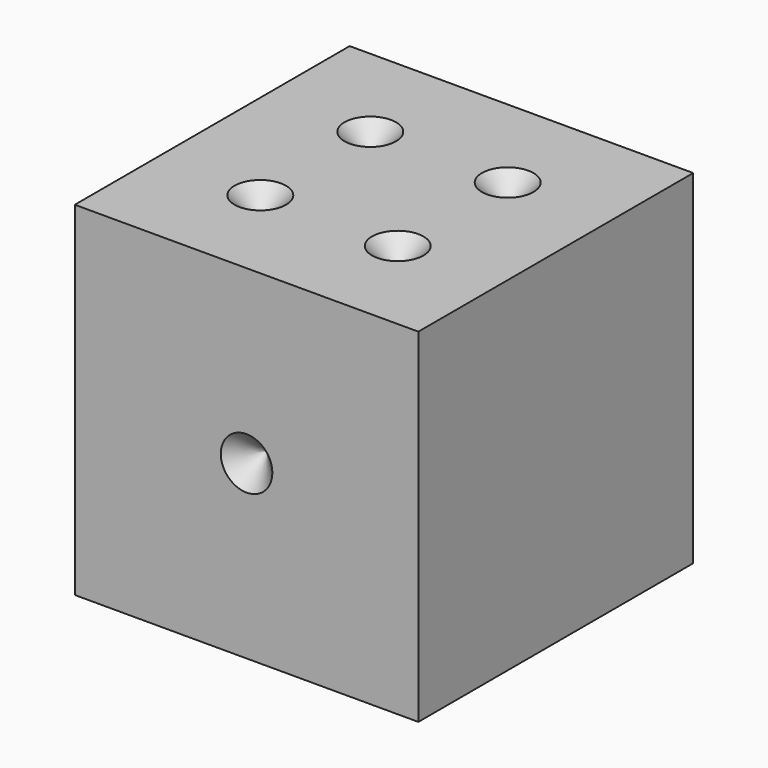
from build123d import *

# Parameters (mm, degrees)
F0_W     = 20
F0_H     = 20
F1_DEPTH = 20
F2_R     = 1.5
F3_DEPTH = 1.5
F4_R     = 1.5
F5_DEPTH = 1.5
F6_SIZE  = 1.49999


# Not quite as in the source:
# - a fillet or chamfer is up to 0.001 mm smaller than in the source, because OpenCascade refuses the exact size


with BuildPart() as f1:
    # F0 (on Top) → F1 (new body)
    with BuildSketch(Plane.XY):
        with Locations((10, 10)):
            Rectangle(F0_W, F0_H)
    extrude(amount=F1_DEPTH)

    # F2 (on face) → F3 (cut)
    with BuildSketch(Plane.XZ):
        with Locations((10, 10)):
            Circle(F2_R)
    extrude(amount=-F3_DEPTH, mode=Mode.SUBTRACT)

    # F4 (on face) → F5 (cut)
    with BuildSketch(Plane.XY.offset(20)):
        with Locations((6, 6)):
            Circle(F4_R)
        with Locations((6, 14)):
            Circle(F4_R)
        with Locations((14, 6)):
            Circle(F4_R)
        with Locations((14, 14)):
            Circle(F4_R)
    extrude(amount=-F5_DEPTH, mode=Mode.SUBTRACT)

    # F6 (size 1.5 in the source; OpenCascade refuses exactly that, so slightly less here)
    f6_edges = [f1.edges().sort_by_distance(p)[0] for p in [
        (8.5, 1.5, 10),
        (4.5, 6, 18.5),
        (4.5, 14, 18.5),
        (12.5, 14, 18.5),
        (12.5, 6, 18.5),
    ]]
    chamfer(f6_edges, length=F6_SIZE)


solid = f1.part
